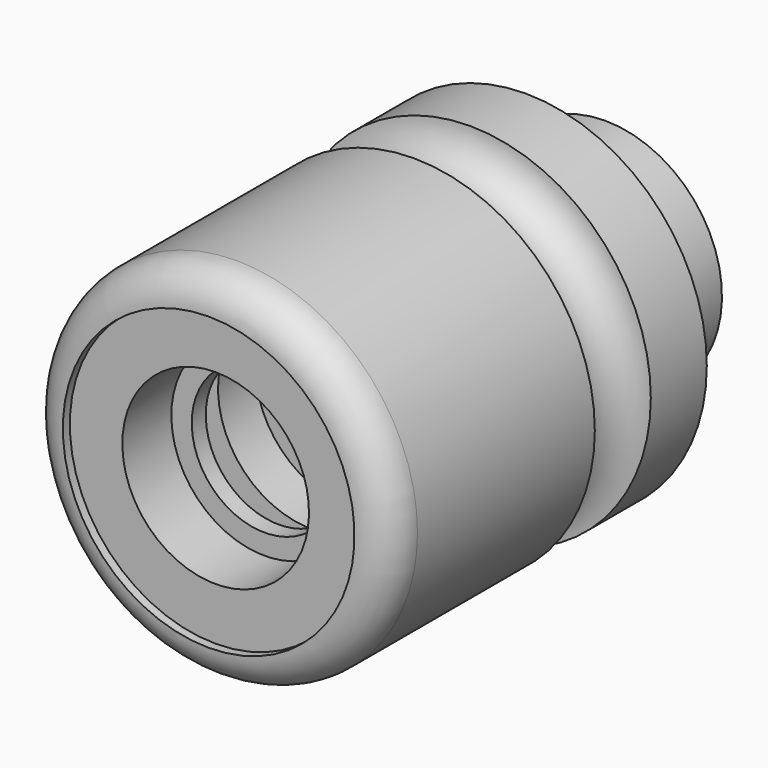
from build123d import *

# Parameters (mm, degrees)
F2_R = 5.99999


# Not quite as in the source:
# - a fillet or chamfer is up to 0.001 mm smaller than in the source, because OpenCascade refuses the exact size


with BuildPart() as f1:
    # F0 (on Right) → F1 (revolve)
    with BuildSketch(Plane.YZ):
        with BuildLine():
            Line((30, 6), (88, 6))
            Line((88, 6), (88, 16))
            Line((88, 16), (85, 16))
            Line((85, 16), (85, 20))
            Line((85, 20), (68, 20))
            Line((68, 20), (68, 31))
            Line((68, 31), (56, 31))
            ThreePointArc((56, 31), (50, 25), (44, 31))
            Line((44, 31), (0, 31))
            Line((0, 31), (0, 25))
            Line((0, 25), (1.5, 25))
            Line((1.5, 25), (1.5, 16))
            Line((1.5, 16), (12, 16))
            Line((12, 16), (12, 12.5))
            Line((12, 12.5), (15, 12.5))
            Line((15, 12.5), (15, 20.5))
            Line((15, 20.5), (22, 20.5))
            Line((22, 20.5), (22, 16))
            Line((22, 16), (30, 16))
            Line((30, 16), (30, 6))
        make_face()
    revolve(axis=Axis((0, 43.1545964642, 0), (0, 1, 0)))

    # F2 (radius 6 in the source; OpenCascade refuses exactly that, so slightly less here)
    f2_edges = [f1.edges().sort_by_distance(p)[0] for p in [
        (0, 0, -31),
    ]]
    fillet(f2_edges, radius=F2_R)


solid = f1.part
